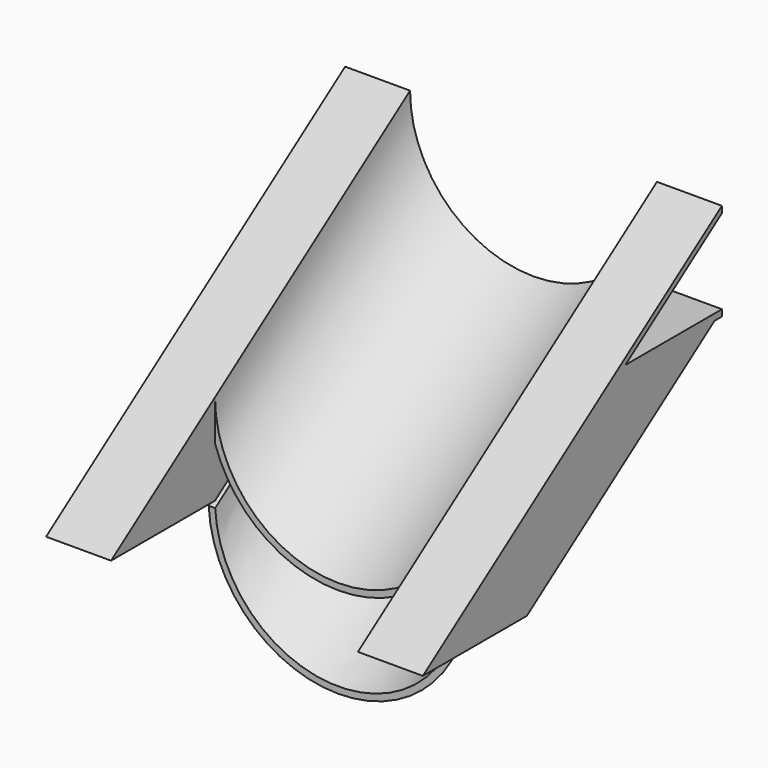
from build123d import *

# Parameters (mm, degrees)
F1_DEPTH  = 25.4
F1_FACE_W = 12.7
F1_FACE_H = 25.4


with BuildPart() as f1:
    # F0 (on Front) → F1 (new body)
    with BuildSketch(Plane.XZ):
        with BuildLine():
            Line((-24.13, 0), (-25.4, 0))
            ThreePointArc((-25.4, 0), (-25.3920562907, -0.6351986549), (-25.3682301314, -1.27))
            Line((-25.3682301314, -1.27), (-24.0965557705, -1.27))
            ThreePointArc((-24.0965557705, -1.27), (-24.1216374936, -0.6352201423), (-24.13, 0))
        make_face()
        with BuildLine():
            ThreePointArc((-25.3682301314, -1.27), (-25.3920562907, -0.6351986549), (-25.4, 0))
            Line((-25.4, 0), (-36.83, 0))
            Line((-36.83, 0), (-36.83, -1.27))
            Line((-36.83, -1.27), (-25.3682301314, -1.27))
        make_face()
        with BuildLine():
            Line((-24.0965557705, -1.27), (-25.3682301314, -1.27))
            ThreePointArc((-25.3682301314, -1.27), (0, -25.4), (25.3682301314, -1.27))
            Line((25.3682301314, -1.27), (24.0965557705, -1.27))
            ThreePointArc((24.0965557705, -1.27), (0, -24.13), (-24.0965557705, -1.27))
        make_face()
        with BuildLine():
            Line((24.0965557705, -1.27), (25.3682301314, -1.27))
            ThreePointArc((25.3682301314, -1.27), (25.3920562907, -0.6351986549), (25.4, 0))
            Line((25.4, 0), (24.13, 0))
            ThreePointArc((24.13, 0), (24.1216374936, -0.6352201423), (24.0965557705, -1.27))
        make_face()
        with BuildLine():
            ThreePointArc((25.4, 0), (25.3920562907, -0.6351986549), (25.3682301314, -1.27))
            Line((25.3682301314, -1.27), (36.83, -1.27))
            Line((36.83, -1.27), (36.83, 0))
            Line((36.83, 0), (25.4, 0))
        make_face()
    extrude(amount=F1_DEPTH)

    # F3: sweep along a path in F2
    with BuildLine(Plane.YZ) as f3_path:
        Line((0, 0), (-47.6711578667, -33.3962440491))
    # F1_face (on face) + F1_face1 (on face) + F0 (on Front) → F3 (sweep)
    with BuildSketch(Plane(origin=(-30.48, -12.7, 0), x_dir=(1, 0, 0), z_dir=(0, 0, 1))):
        Rectangle(F1_FACE_W, F1_FACE_H)
        with Locations((60.96, 0)):
            Rectangle(F1_FACE_W, F1_FACE_H)
    with BuildSketch(Plane(origin=(1e-10, -25.4, -12.329976557), x_dir=(1, 0, 0), z_dir=(0, -1, 0))):
        with BuildLine():
            Line((-24.1300000001, 12.329976557), (-36.8300000001, 12.329976557))
            Line((-36.8300000001, 12.329976557), (-36.8300000001, 11.059976557))
            Line((-36.8300000001, 11.059976557), (-25.3682301315, 11.059976557))
            ThreePointArc((-25.3682301315, 11.059976557), (-1e-10, -13.070023443), (25.3682301313, 11.059976557))
            Line((25.3682301313, 11.059976557), (36.8299999999, 11.059976557))
            Line((36.8299999999, 11.059976557), (36.8299999999, 12.329976557))
            Line((36.8299999999, 12.329976557), (24.1299999999, 12.329976557))
            ThreePointArc((24.1299999999, 12.329976557), (-1e-10, -11.8000234431), (-24.1300000001, 12.329976557))
        make_face()
    with BuildSketch(Plane.XZ):
        with BuildLine():
            Line((-24.0965557705, -1.27), (-25.3682301314, -1.27))
            ThreePointArc((-25.3682301314, -1.27), (0, -25.4), (25.3682301314, -1.27))
            Line((25.3682301314, -1.27), (24.0965557705, -1.27))
            ThreePointArc((24.0965557705, -1.27), (0, -24.13), (-24.0965557705, -1.27))
        make_face()
    sweep(path=f3_path.line)


solid = f1.part
